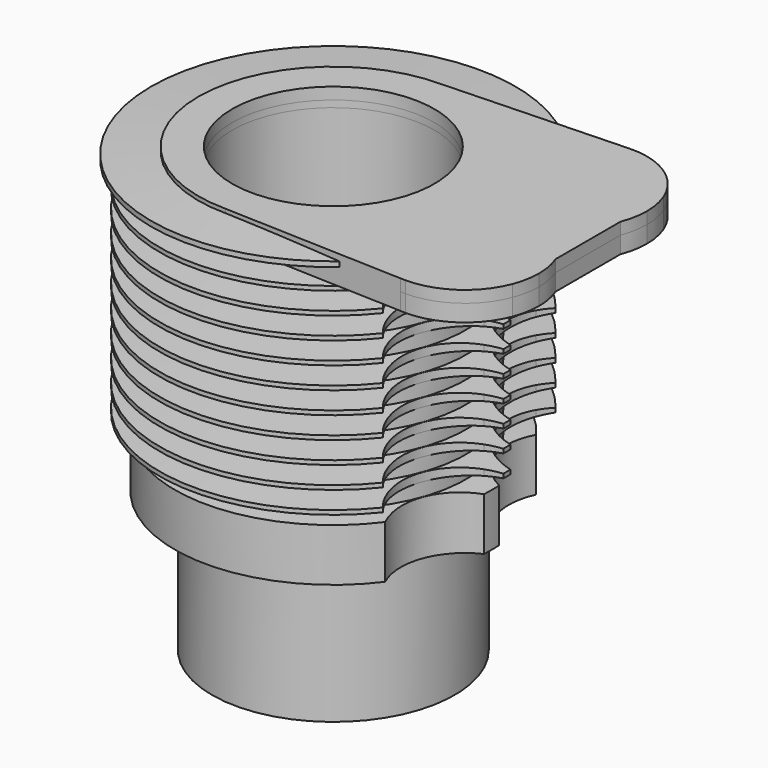
from build123d import *

# Parameters (mm, degrees)
F5_DEPTH  = 200
F9_DEPTH  = 10
F10_DEPTH = 7


with BuildPart() as f1:
    # F0 (on Front) → F1 (revolve)
    with BuildSketch(Plane.XZ):
        Polygon((-60, -252), (-60, 0), (-65, 0), (-74, 0), (-74, -7), (-73, -7), (-73, -169), (-72, -169), (-72, -252), align=None)
    revolve(axis=Axis((0, 0, -33.1248603761), (0, 0, -1)))


with BuildPart() as f3:
    # F2 (on Front) → F3 (revolve)
    with BuildSketch(Plane.XZ):
        Polygon((-94, -169), (-79, -169), (-79, -142.0155734056), (-94, -141.2294567163), align=None)
        Polygon((-73, -169), (-73, -7), (-79, -7), (-79, -12.0155734056), (-79, -20), (-79, -25.0155734056), (-79, -33), (-79, -38.0155734056), (-79, -46), (-79, -51.0155734056), (-79, -59), (-79, -64.0155734056), (-79, -72), (-79, -77.0155734056), (-79, -85), (-79, -90.0155734056), (-79, -98), (-79, -103.0155734056), (-79, -111), (-79, -116.0155734056), (-79, -124), (-79, -129.0155734056), (-79, -137), (-79, -139.0155734056), (-79, -142.0155734056), (-79, -169), align=None)
        Polygon((-103, -127.7577867028), (-79, -129.0155734056), (-79, -124), (-103, -125.2577867028), align=None)
        Polygon((-103, -114.7577867028), (-79, -116.0155734056), (-79, -111), (-103, -112.2577867028), align=None)
        Polygon((-103, -101.7577867028), (-79, -103.0155734056), (-79, -98), (-103, -99.2577867028), align=None)
        Polygon((-103, -88.7577867028), (-79, -90.0155734056), (-79, -85), (-103, -86.2577867028), align=None)
        Polygon((-79, -77.0155734056), (-79, -72), (-103, -73.2577867028), (-103, -75.7577867028), align=None)
        Polygon((-79, -64.0155734056), (-79, -59), (-103, -60.2577867028), (-103, -62.7577867028), align=None)
        Polygon((-79, -51.0155734056), (-79, -46), (-103, -47.2577867028), (-103, -49.7577867028), align=None)
        Polygon((-79, -38.0155734056), (-79, -33), (-103, -34.2577867028), (-103, -36.7577867028), align=None)
        Polygon((-79, -25.0155734056), (-79, -20), (-103, -21.2577867028), (-103, -23.7577867028), align=None)
        Polygon((-79, -12.0155734056), (-79, -7), (-103, -8.2577867028), (-103, -10.7577867028), align=None)
        Polygon((-94, -139.0155734056), (-79, -139.0155734056), (-79, -137), (-94, -137.7861166892), align=None)
        Polygon((-94, -141.2294567163), (-79, -142.0155734056), (-79, -139.0155734056), (-94, -139.0155734056), align=None)
    revolve(axis=Axis((0, 0, -33.1248603761), (0, 0, -1)))

    # F4 (on face) → F5 (cut)
    with BuildSketch(Plane(origin=(0, 0, -169), x_dir=(1, 0, 0), z_dir=(0, 0, -1))):
        with BuildLine():
            ThreePointArc((93.8323905069, 5.6109261061), (130.3670179366, 7.9190932115), (148, 40))
            ThreePointArc((148, 40), (118.1773621604, 77.1097123149), (75.5194343107, 55.9715556457))
            ThreePointArc((75.5194343107, 55.9715556457), (88.3405818079, 32.1238479302), (93.8323905069, 5.6109261061))
        make_face()
        with BuildLine():
            ThreePointArc((93.8323905069, -5.6109261061), (88.3405818079, -32.1238479301), (75.5194343107, -55.9715556457))
            ThreePointArc((75.5194343107, -55.9715556457), (118.1773621604, -77.1097123149), (148, -40))
            ThreePointArc((148, -40), (130.3670179366, -7.9190932115), (93.8323905069, -5.6109261061))
        make_face()
        with BuildLine():
            ThreePointArc((93.8323905069, 5.6109261061), (88.3405818079, 32.1238479302), (75.5194343107, 55.9715556457))
            ThreePointArc((75.5194343107, 55.9715556457), (74.2878499074, 27.0137636027), (93.8323905069, 5.6109261061))
        make_face()
        with BuildLine():
            ThreePointArc((93.8323905069, -5.6109261061), (74.2878499074, -27.0137636027), (75.5194343107, -55.9715556457))
            ThreePointArc((75.5194343107, -55.9715556457), (88.3405818079, -32.1238479301), (93.8323905069, -5.6109261061))
        make_face()
    extrude(amount=-F5_DEPTH, mode=Mode.SUBTRACT)


with BuildPart() as f7:
    # F6 (on Front) → F7 (revolve)
    with BuildSketch(Plane.XZ):
        Polygon((-74, 0), (-60, 0), (-60, 4), (-80, 4), (-80, -6), (-74, -6), align=None)
    revolve(axis=Axis((0, 0, -33.1248603761), (0, 0, -1)))

    # F8 (on face) → F9 (join)
    with BuildSketch(Plane.XY.offset(4)):
        with BuildLine():
            ThreePointArc((110, -84), (134.8332070563, -76.3223323494), (151, -55.9687194227))
            Line((151, -55.9687194227), (151, -24.0312805773))
            ThreePointArc((151, -24.0312805773), (142.006199689, -9.8072329611), (128.3303027798, 0))
            ThreePointArc((128.3303027798, 0), (110, -4), (91.6696972202, 0))
            ThreePointArc((91.6696972202, 0), (85.2801322902, -3.6004376343), (79.5773824685, -8.2121982117))
            ThreePointArc((79.5773824685, -8.2121982117), (75.1834738791, -27.3394450469), (66.264953298, -44.8213784306))
            ThreePointArc((66.264953298, -44.8213784306), (79.4697938556, -71.6844837859), (106.8042258171, -83.8837900297))
            Line((106.8042258171, -83.8837900297), (110, -84))
        make_face()
        with BuildLine():
            Line((151, -24.0312805773), (151, -55.9687194227))
            ThreePointArc((151, -55.9687194227), (153.2434966209, -48.1240384046), (154, -40))
            ThreePointArc((154, -40), (153.2434966209, -31.8759615954), (151, -24.0312805773))
        make_face()
        with BuildLine():
            ThreePointArc((128.3303027798, 0), (142.006199689, -9.8072329611), (151, -24.0312805773))
            Line((151, -24.0312805773), (151, 24.0312805773))
            ThreePointArc((151, 24.0312805773), (142.006199689, 9.8072329611), (128.3303027798, 0))
        make_face()
        with BuildLine():
            ThreePointArc((128.3303027798, 0), (142.006199689, 9.8072329611), (151, 24.0312805773))
            Line((151, 24.0312805773), (151, 55.9687194227))
            ThreePointArc((151, 55.9687194227), (134.1641022949, 76.7708602059), (108.3892776713, 83.9705079977))
            ThreePointArc((108.3892776713, 83.9705079977), (80.0463144386, 72.2300592815), (66.264953298, 44.8213784306))
            ThreePointArc((66.264953298, 44.8213784306), (75.1834738791, 27.3394450469), (79.5773824685, 8.2121982117))
            ThreePointArc((79.5773824685, 8.2121982117), (85.2801322902, 3.6004376343), (91.6696972202, 0))
            ThreePointArc((91.6696972202, 0), (110, 4), (128.3303027798, 0))
        make_face()
        with BuildLine():
            Line((151, 55.9687194227), (151, 24.0312805773))
            ThreePointArc((151, 24.0312805773), (153.2434966209, 31.8759615954), (154, 40))
            ThreePointArc((154, 40), (153.2434966209, 48.1240384046), (151, 55.9687194227))
        make_face()
        with BuildLine():
            ThreePointArc((91.6696972202, 0), (110, -4), (128.3303027798, 0))
            ThreePointArc((128.3303027798, 0), (110, 4), (91.6696972202, 0))
        make_face()
        with BuildLine():
            Line((0, -80), (106.8042258171, -83.8837900297))
            ThreePointArc((106.8042258171, -83.8837900297), (79.4697938556, -71.6844837859), (66.264953298, -44.8213784306))
            ThreePointArc((66.264953298, -44.8213784306), (37.5119296061, -70.660138248), (0, -80))
        make_face()
        with BuildLine():
            ThreePointArc((79.5773824685, -8.2121982117), (85.2801322902, -3.6004376343), (91.6696972202, 0))
            ThreePointArc((91.6696972202, 0), (85.2801322902, 3.6004376343), (79.5773824685, 8.2121982117))
            ThreePointArc((79.5773824685, 8.2121982117), (79.894275757, 4.1115327144), (80, 0))
            ThreePointArc((80, 0), (79.894275757, -4.1115327144), (79.5773824685, -8.2121982117))
        make_face()
        with BuildLine():
            ThreePointArc((66.264953298, 44.8213784306), (80.0463144386, 72.2300592815), (108.3892776713, 83.9705079977))
            Line((108.3892776713, 83.9705079977), (0, 80))
            ThreePointArc((0, 80), (37.5119296061, 70.660138248), (66.264953298, 44.8213784306))
        make_face()
    extrude(amount=-F9_DEPTH)

    # F10 (add): a face of the model
    f10_faces = [f7.faces().sort_by_distance(p)[0] for p in [
        (64.2280615389, 0.0057342753, 4),
    ]]
    extrude(f10_faces, amount=F10_DEPTH)

    # F11 (on Front) → F12 (revolve)
    with BuildSketch(Plane.XZ):
        Polygon((-108, 7.1819318197), (-108, 4.1819318197), (-73.3091925435, 2.3638636393), (-73.3091925435, 9), align=None)
    revolve(axis=Axis((0, 0, -33.1248603761), (0, 0, -1)))


solid = Compound([f1.part, f3.part, f7.part])
